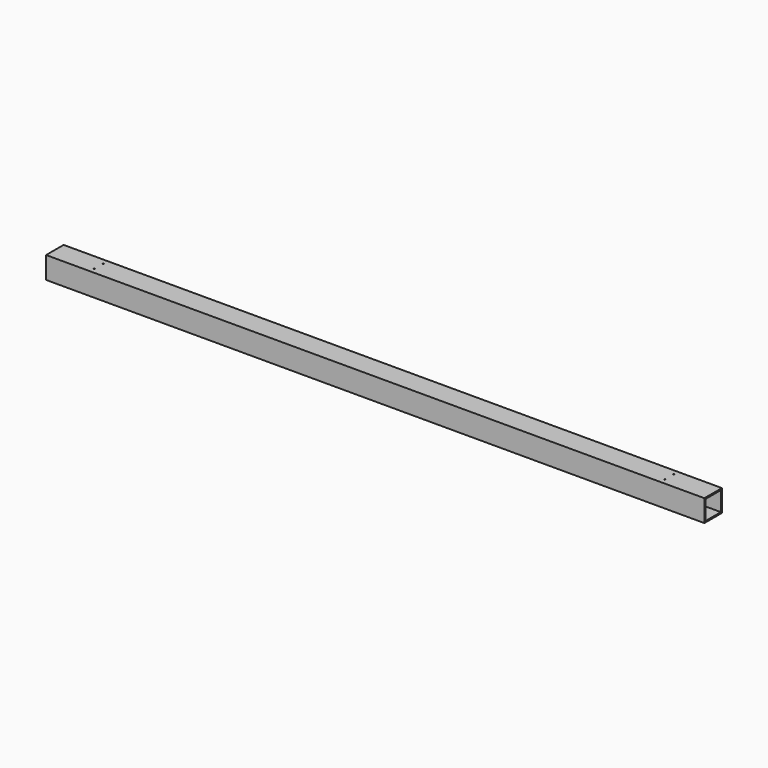
from build123d import *

# Parameters (mm, degrees)
F0_W     = 101.6
F0_H     = 101.6
F0_W_2   = 89.5604
F0_H_2   = 89.5604
F1_DEPTH = 1524
F3_D     = 5.1054


with BuildPart() as f1:
    # F0 (on Right) → F1 (new body, symmetric)
    with BuildSketch(Plane.YZ):
        Rectangle(F0_W, F0_H)
        Rectangle(F0_W_2, F0_H_2, mode=Mode.SUBTRACT)
    extrude(amount=F1_DEPTH, both=True)

    # F3 (through all)
    with Locations(Plane.XY.offset(50.8)):
        with Locations((-1320.8, 25.4), (-1320.8, -25.4), (1320.8, 25.4), (1320.8, -25.4)):
            Hole(F3_D / 2)


solid = f1.part
